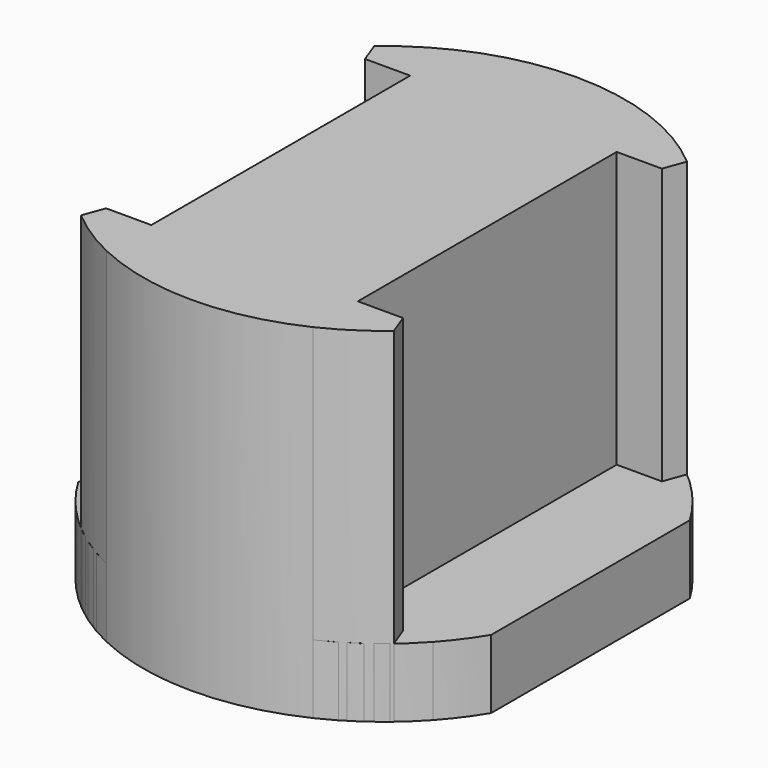
from build123d import *

# Parameters (mm, degrees)
F1_DEPTH    = 5
F0_W        = 15
F0_H        = 23.5
F0_R        = 3.5
F2_DEPTH    = 25
F3_T1_DEPTH = 36.3750267574
F4_DEPTH    = 15


# Not quite as in the source:
# - a fillet or chamfer that OpenCascade refuses, or shapes differently, is made with other operations: its cross-section is extruded or revolved along the edge and cut away or added
# - a feature names something its author has since deleted; it is built from what else it names


with BuildPart() as f1:
    # F0 (on Top) → F1 (new body)
    with BuildSketch(Plane.XY):
        with BuildLine():
            Line((15, -9.0138781887), (15, 9.0138781887))
            ThreePointArc((15, 9.0138781887), (14.0511141288, 10.4314999755), (12.9687123493, 11.75))
            Line((12.9687123493, 11.75), (7.5, 11.75))
            Line((7.5, 11.75), (7.5, -11.75))
            Line((7.5, -11.75), (12.9687123493, -11.75))
            ThreePointArc((12.9687123493, -11.75), (14.0511141288, -10.4314999755), (15, -9.0138781887))
        make_face()
        with BuildLine():
            ThreePointArc((7.5, -15.8113883008), (10.4338758399, -14.0493499834), (12.9687123493, -11.75))
            Line((12.9687123493, -11.75), (7.5, -11.75))
            Line((7.5, -11.75), (7.5, -15.8113883008))
        make_face()
        with BuildLine():
            Line((7.5, 11.75), (12.9687123493, 11.75))
            ThreePointArc((12.9687123493, 11.75), (10.4338758399, 14.0493499834), (7.5, 15.8113883008))
            Line((7.5, 15.8113883008), (7.5, 11.75))
        make_face()
    extrude(amount=F1_DEPTH)


with BuildPart() as f1b:
    # F0 (on Top) → F1, piece 2 (new body)
    with BuildSketch(Plane.XY):
        with BuildLine():
            Line((-7.5, -11.75), (-7.5, 11.75))
            Line((-7.5, 11.75), (-12.9687123493, 11.75))
            ThreePointArc((-12.9687123493, 11.75), (-14.0511141288, 10.4314999755), (-15, 9.0138781887))
            Line((-15, 9.0138781887), (-15, -9.0138781887))
            ThreePointArc((-15, -9.0138781887), (-14.0511141288, -10.4314999755), (-12.9687123493, -11.75))
            Line((-12.9687123493, -11.75), (-7.5, -11.75))
        make_face()
        with BuildLine():
            Line((-7.5, 11.75), (-7.5, 15.8113883008))
            ThreePointArc((-7.5, 15.8113883008), (-10.4338758399, 14.0493499834), (-12.9687123493, 11.75))
            Line((-12.9687123493, 11.75), (-7.5, 11.75))
        make_face()
        with BuildLine():
            ThreePointArc((-12.9687123493, -11.75), (-10.4338758399, -14.0493499834), (-7.5, -15.8113883008))
            Line((-7.5, -15.8113883008), (-7.5, -11.75))
            Line((-7.5, -11.75), (-12.9687123493, -11.75))
        make_face()
    extrude(amount=F1_DEPTH)


with BuildPart() as f2:
    # F0 (on Top) → F2 (new body)
    with BuildSketch(Plane.XY):
        Rectangle(F0_W, F0_H)
        Circle(F0_R, mode=Mode.SUBTRACT)
        with BuildLine():
            ThreePointArc((-12.9687123493, -11.75), (-10.4338758399, -14.0493499834), (-7.5, -15.8113883008))
            Line((-7.5, -15.8113883008), (-7.5, -11.75))
            Line((-7.5, -11.75), (-12.9687123493, -11.75))
        make_face()
        with BuildLine():
            Line((-7.5, 11.75), (-7.5, 15.8113883008))
            ThreePointArc((-7.5, 15.8113883008), (-10.4338758399, 14.0493499834), (-12.9687123493, 11.75))
            Line((-12.9687123493, 11.75), (-7.5, 11.75))
        make_face()
        with BuildLine():
            Line((7.5, 11.75), (12.9687123493, 11.75))
            ThreePointArc((12.9687123493, 11.75), (10.4338758399, 14.0493499834), (7.5, 15.8113883008))
            Line((7.5, 15.8113883008), (7.5, 11.75))
        make_face()
        with BuildLine():
            ThreePointArc((7.5, -15.8113883008), (10.4338758399, -14.0493499834), (12.9687123493, -11.75))
            Line((12.9687123493, -11.75), (7.5, -11.75))
            Line((7.5, -11.75), (7.5, -15.8113883008))
        make_face()
        with BuildLine():
            Line((7.5, 11.75), (7.5, 15.8113883008))
            ThreePointArc((7.5, 15.8113883008), (0, 17.5), (-7.5, 15.8113883008))
            Line((-7.5, 15.8113883008), (-7.5, 11.75))
            Line((-7.5, 11.75), (7.5, 11.75))
        make_face()
        with BuildLine():
            ThreePointArc((-7.5, -15.8113883008), (0, -17.5), (7.5, -15.8113883008))
            Line((7.5, -15.8113883008), (7.5, -11.75))
            Line((7.5, -11.75), (-7.5, -11.75))
            Line((-7.5, -11.75), (-7.5, -15.8113883008))
        make_face()
        Circle(F0_R)
    extrude(amount=F2_DEPTH)

    # F3: chamfer of 2 on 4 edges, made by hand

    # F3_s2 → F3_t1 (cut)
    with BuildSketch(Plane.XY.offset(-5.6875133787)):
        with BuildLine():
            Line((-10.7571586121, -11.6749396443), (-11.3881617362, -13.3863096005))
            Line((-11.3881617362, -13.3863096005), (-11.4141285615, -13.4167353131))
            ThreePointArc((-11.4141285615, -13.4167353131), (-12.2058182488, -12.5964122224), (-12.9983551204, -11.7768571429))
            Line((-12.9983551204, -11.7768571429), (-12.9687123493, -11.71))
            ThreePointArc((-12.9687123493, -11.71), (-11.8629354807, -11.71), (-10.7571586121, -11.6349396443))
            Line((-10.7571586121, -11.6349396443), (-10.7571586121, -11.6749396443))
        make_face()
        with BuildLine():
            Line((11.3881617362, -13.3863096005), (10.7571586121, -11.6749396443))
            Line((10.7571586121, -11.6749396443), (10.7571586121, -11.6349396443))
            ThreePointArc((10.7571586121, -11.6349396443), (11.8629354807, -11.71), (12.9687123493, -11.71))
            Line((12.9687123493, -11.71), (12.9983551204, -11.7768571429))
            ThreePointArc((12.9983551204, -11.7768571429), (12.2058182488, -12.5964122224), (11.4141285615, -13.4167353131))
            Line((11.4141285615, -13.4167353131), (11.3881617362, -13.3863096005))
        make_face()
        with BuildLine():
            Line((10.7571586121, 11.6749396443), (11.3881617362, 13.3863096005))
            Line((11.3881617362, 13.3863096005), (11.4141285615, 13.4167353131))
            ThreePointArc((11.4141285615, 13.4167353131), (12.2058182488, 12.5964122224), (12.9983551204, 11.7768571429))
            Line((12.9983551204, 11.7768571429), (12.9687123493, 11.71))
            ThreePointArc((12.9687123493, 11.71), (11.8629354807, 11.71), (10.7571586121, 11.6349396443))
            Line((10.7571586121, 11.6349396443), (10.7571586121, 11.6749396443))
        make_face()
        with BuildLine():
            Line((-11.3881617362, 13.3863096005), (-10.7571586121, 11.6749396443))
            Line((-10.7571586121, 11.6749396443), (-10.7571586121, 11.6349396443))
            ThreePointArc((-10.7571586121, 11.6349396443), (-11.8629354807, 11.71), (-12.9687123493, 11.71))
            Line((-12.9687123493, 11.71), (-12.9983551204, 11.7768571429))
            ThreePointArc((-12.9983551204, 11.7768571429), (-12.2058182488, 12.5964122224), (-11.4141285615, 13.4167353131))
            Line((-11.4141285615, 13.4167353131), (-11.3881617362, 13.3863096005))
        make_face()
    extrude(amount=F3_T1_DEPTH, mode=Mode.SUBTRACT)

    # F0 (on Top) → F4 (cut)
    with BuildSketch(Plane.XY):
        Circle(F0_R)
    extrude(amount=F4_DEPTH, mode=Mode.SUBTRACT)


solid = Compound([f1.part, f1b.part, f2.part])
